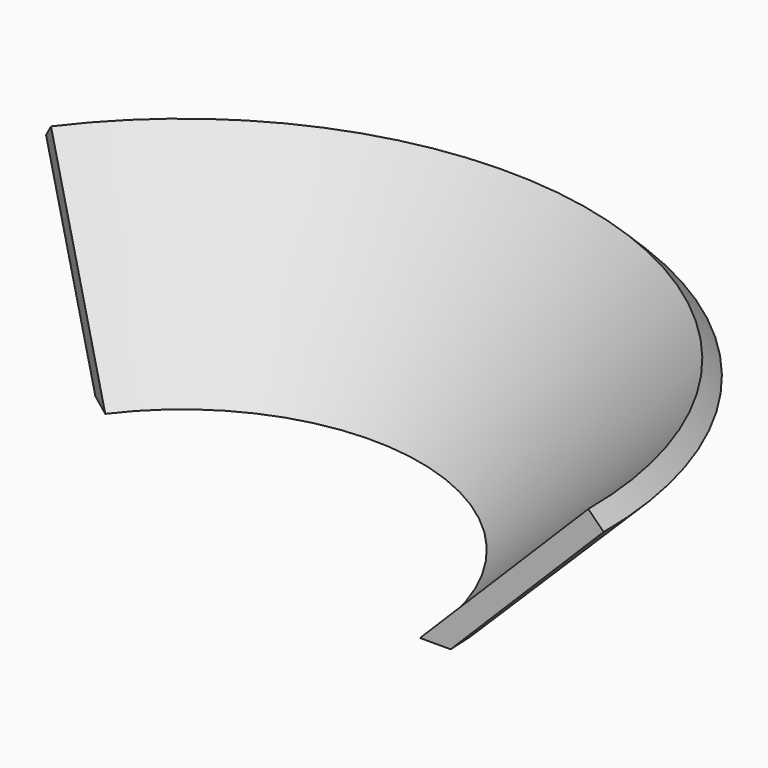
from build123d import *

# Parameters (mm, degrees)
F1_ANGLE = 143.2394
F2_SCALE = 10


# Not quite as in the source:
# - a feature names something its author has since deleted; it is built from what else it names


with BuildPart() as f1:
    # F0 (on Front) → F1 (revolve)
    with BuildSketch(Plane.XZ):
        Polygon((24.8284271247, 1.4142135624), (38.9705627485, 15.5563491861), (37.5563491861, 16.9705627485), (22, 1.4142135624), align=None)
    revolve(axis=Axis((0, 0, 11), (0, 0, 1)), revolution_arc=F1_ANGLE)


with BuildPart() as f1_1:
    # F2: moved
    add(f1.part.scale(F2_SCALE).moved(Location((-338.0071426749, 0, -152.7350647363))))


solid = f1_1.part
